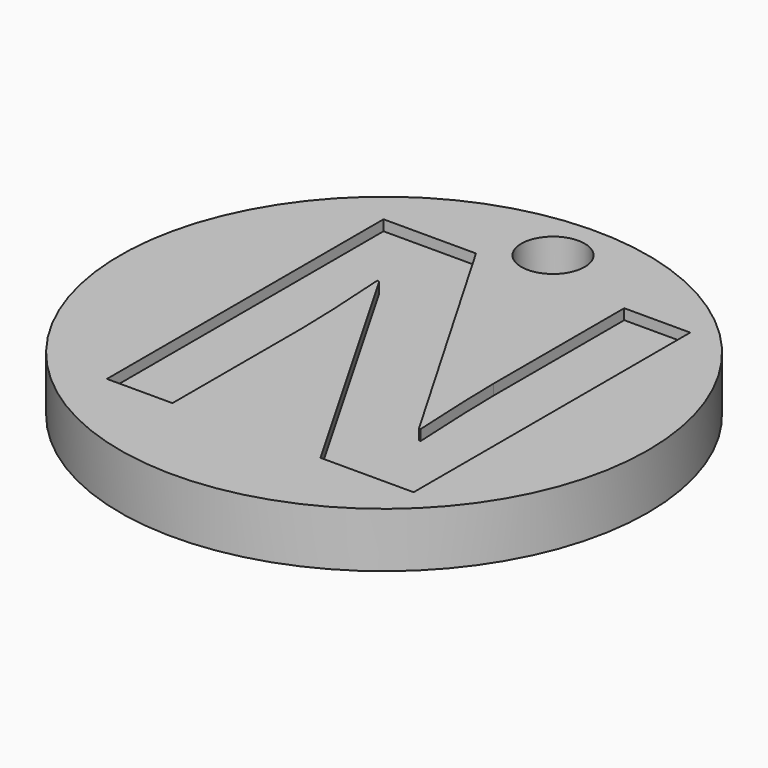
from build123d import *

# Parameters (mm, degrees)
F0_R         = 12.5
F1_DEPTH     = 2.6
F2_TEXT_SIZE = 22.9347031564
F3_DEPTH     = 0.5
F4_R         = 1.5
F5_DEPTH     = 25


# Not quite as in the source:
# - Text() gives the source's letters only with a copy of the font that has no kerning and outlines rounded to 1/6400 em; it was checked with that copy


with BuildPart() as f1:
    # F0 (on Top) → F1 (new body)
    with BuildSketch(Plane.XY):
        Circle(F0_R)
    extrude(amount=F1_DEPTH)

    # F2 (on face) → F3 (cut)
    with BuildSketch(Plane.XY.offset(2.6)):
        with Locations((-8.756105497, -8.0374069512)):
            Text('N', F2_TEXT_SIZE, font='Open Sans', font_style=FontStyle.BOLD, text_align=(TextAlign.LEFT, TextAlign.BOTTOM))
    extrude(amount=-F3_DEPTH, mode=Mode.SUBTRACT)

    # F4 (on face) → F5 (cut)
    with BuildSketch(Plane.XY.offset(2.6)):
        with Locations((0, 10)):
            Circle(F4_R)
    extrude(amount=-F5_DEPTH, mode=Mode.SUBTRACT)


solid = f1.part
